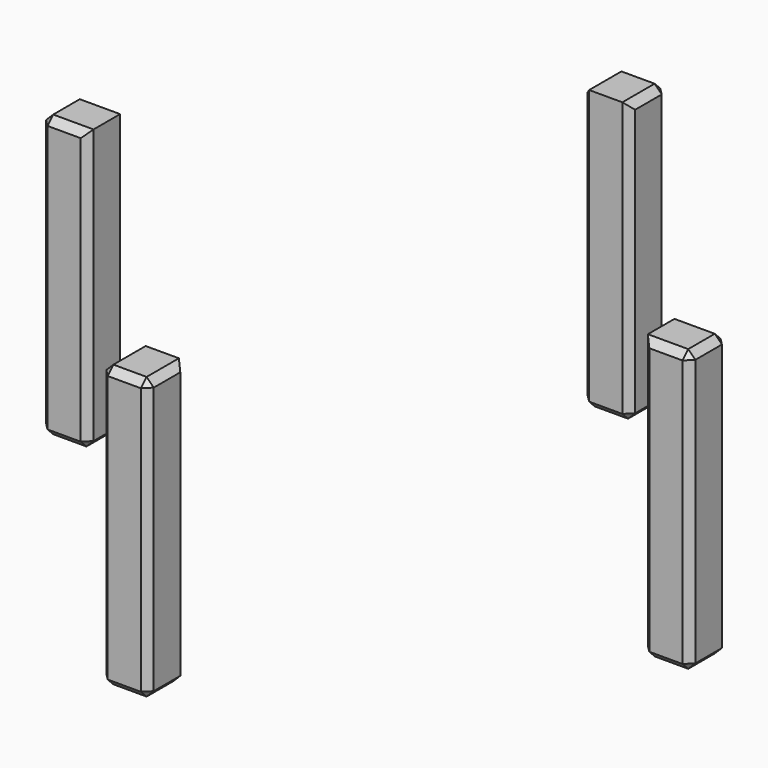
from build123d import *

# Parameters (mm, degrees)
F4_DEPTH        = 500
F4_DEPTH_BACK   = 93
F4_COPIES_COUNT = 4
F5_SIZE         = 15
F5_2_SIZE       = 15
F5_3_SIZE       = 15
F5_4_SIZE       = 15


# Not quite as in the source:
# - a feature of the source that left no trace in its solid (it failed there, or was rolled back) is left out
# - a pattern or mirror of a feature is missing from the dataset's text; its kind, count and spacing are read off the source's solid
# - the program builds the solid bodies; features that only make, move or delete a surface that nothing else refers to are left out


with BuildPart() as f4:
    # F3 (on offset) → F4 (new body, two sides)
    with BuildSketch(Plane.XY.offset(550)) as f4_sk:
        with BuildLine():
            Line((50, -584), (-50, -584))
            Line((-50, -584), (-50, -632.0253159487))
            ThreePointArc((-50, -632.0253159487), (0, -634), (50, -632.0253159487))
            Line((50, -632.0253159487), (50, -584))
        make_face()
        with BuildLine():
            ThreePointArc((50, -632.0253159487), (0, -634), (-50, -632.0253159487))
            Line((-50, -632.0253159487), (-50, -684))
            Line((-50, -684), (50, -684))
            Line((50, -684), (50, -632.0253159487))
        make_face()
    extrude(amount=-F4_DEPTH)
    extrude(f4_sk.sketch, amount=F4_DEPTH_BACK)


with BuildPart() as f4_copies_1:
    # F4_copies: instance of F4
    add(f4.part.rotate(Axis((0, 0, 0), (0, 0, 1)), 1 * 360 / F4_COPIES_COUNT))

    # F5#2
    f5_2_edges = [f4_copies_1.edges().sort_by_distance(p)[0] for p in [
        (584, 0, 50),
        (584, -50, 346.5),
        (584, 50, 346.5),
        (634, 50, 50),
        (634, 50, 643),
        (684, 50, 346.5),
        (684, -50, 346.5),
        (684, 0, 50),
        (684, 0, 643),
        (634, -50, 643),
        (634, -50, 50),
    ]]
    chamfer(f5_2_edges, length=F5_2_SIZE)


with BuildPart() as f4_copies_2:
    # F4_copies: instance of F4
    add(f4.part.rotate(Axis((0, 0, 0), (0, 0, 1)), 2 * 360 / F4_COPIES_COUNT))

    # F5#3
    f5_3_edges = [f4_copies_2.edges().sort_by_distance(p)[0] for p in [
        (0, 584, 50),
        (50, 584, 346.5),
        (-50, 584, 346.5),
        (-50, 634, 50),
        (-50, 634, 643),
        (-50, 684, 346.5),
        (50, 684, 346.5),
        (0, 684, 50),
        (0, 684, 643),
        (50, 634, 643),
        (50, 634, 50),
    ]]
    chamfer(f5_3_edges, length=F5_3_SIZE)


with BuildPart() as f4_copies_3:
    # F4_copies: instance of F4
    add(f4.part.rotate(Axis((0, 0, 0), (0, 0, 1)), 3 * 360 / F4_COPIES_COUNT))

    # F5#4
    f5_4_edges = [f4_copies_3.edges().sort_by_distance(p)[0] for p in [
        (-584, 0, 50),
        (-584, 50, 346.5),
        (-584, -50, 346.5),
        (-634, -50, 50),
        (-634, -50, 643),
        (-684, -50, 346.5),
        (-684, 50, 346.5),
        (-684, 0, 50),
        (-684, 0, 643),
        (-634, 50, 643),
        (-634, 50, 50),
    ]]
    chamfer(f5_4_edges, length=F5_4_SIZE)


with BuildPart() as f4_1:
    add(f4.part)

    # F5
    f5_edges = [f4_1.edges().sort_by_distance(p)[0] for p in [
        (50, -684, 346.5),
        (50, -634, 643),
        (0, -684, 643),
        (-50, -634, 643),
        (50, -584, 346.5),
        (-50, -584, 346.5),
        (-50, -684, 346.5),
        (0, -684, 50),
        (-50, -634, 50),
        (0, -584, 50),
        (50, -634, 50),
    ]]
    chamfer(f5_edges, length=F5_SIZE)


solid = Compound([f4_copies_1.part, f4_copies_2.part, f4_copies_3.part, f4_1.part])
